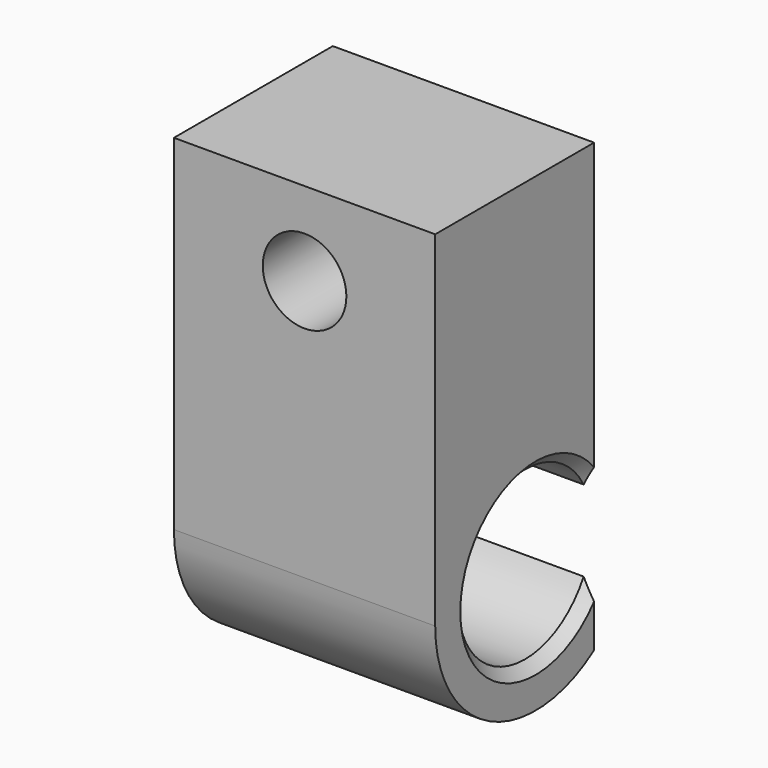
from build123d import *

# Parameters (mm, degrees)
F1_DEPTH = 25
F3_W     = 25
F3_H     = 33
F3_H_2   = 17
F4_DEPTH = 5
F6_DEPTH = 25


# Not quite as in the source:
# - a fillet or chamfer that OpenCascade refuses, or shapes differently, is made with other operations: its cross-section is extruded or revolved along the edge and cut away or added


with BuildPart() as f1:
    # F0 (on Right) → F1 (new body)
    with BuildSketch(Plane.YZ):
        with BuildLine():
            ThreePointArc((0, 8), (5.6568542495, 5.6568542495), (8, 0))
            Line((8, 0), (12, 0))
            ThreePointArc((12, 0), (8.4852813742, 8.4852813742), (0, 12))
            Line((0, 12), (0, 8))
        make_face()
        with BuildLine():
            Line((12, 0), (8, 0))
            ThreePointArc((8, 0), (0, -8), (-8, 0))
            Line((-8, 0), (-12, 0))
            ThreePointArc((-12, 0), (0, -12), (12, 0))
        make_face()
        with BuildLine():
            ThreePointArc((-8, 0), (-5.6568542495, 5.6568542495), (0, 8))
            Line((0, 8), (0, 12))
            ThreePointArc((0, 12), (-8.4852813742, 8.4852813742), (-12, 0))
            Line((-12, 0), (-8, 0))
        make_face()
        with BuildLine():
            ThreePointArc((-12, 0), (-8.4852813742, 8.4852813742), (0, 12))
            Line((0, 12), (0, 25))
            Line((0, 25), (0, 29))
            Line((0, 29), (0, 33))
            Line((0, 33), (-12, 33))
            Line((-12, 33), (-12, 0))
        make_face()
        with BuildLine():
            ThreePointArc((0, 12), (8.4852813742, 8.4852813742), (12, 0))
            Line((12, 0), (12, 33))
            Line((12, 33), (0, 33))
            Line((0, 33), (0, 29))
            Line((0, 29), (0, 25))
            Line((0, 25), (0, 12))
        make_face()
    extrude(amount=F1_DEPTH)

    # F2: chamfer of 1 on 2 edges, made by hand

    # F2_s1 → F2_t2 (revolve, cut)
    with BuildSketch(Plane.XY):
        Polygon((24, -8), (25, -9), (25, -8), align=None)
    revolve(axis=Axis((25, 0, 0), (-1, 0, 0)), mode=Mode.SUBTRACT)

    # F2_s3 → F2_t4 (revolve, cut)
    with BuildSketch(Plane.XY):
        Polygon((1, -8), (0, -9), (0, -8), align=None)
    revolve(axis=Axis((0, 0, 0), (-1, 0, 0)), mode=Mode.SUBTRACT)

    # F3 (on face) → F4 (cut)
    with BuildSketch(Plane(origin=(0, 12, 0), x_dir=(-1, 0, 0), z_dir=(0, 1, 0))):
        with Locations((-12.5, 16.5)):
            Rectangle(F3_W, F3_H)
        with Locations((-12.5, -8.5)):
            Rectangle(F3_W, F3_H_2)
    extrude(amount=-F4_DEPTH, mode=Mode.SUBTRACT)

    # F5 (on face) → F6 (cut)
    with BuildSketch(Plane.XZ.offset(12)):
        with BuildLine():
            Line((12.5, 25), (8.5, 25))
            ThreePointArc((8.5, 25), (12.5, 21), (16.5, 25))
            Line((16.5, 25), (12.5, 25))
        make_face()
        with BuildLine():
            ThreePointArc((16.5, 25), (12.5, 29), (8.5, 25))
            Line((8.5, 25), (12.5, 25))
            Line((12.5, 25), (16.5, 25))
        make_face()
    extrude(amount=-F6_DEPTH, mode=Mode.SUBTRACT)


solid = f1.part
